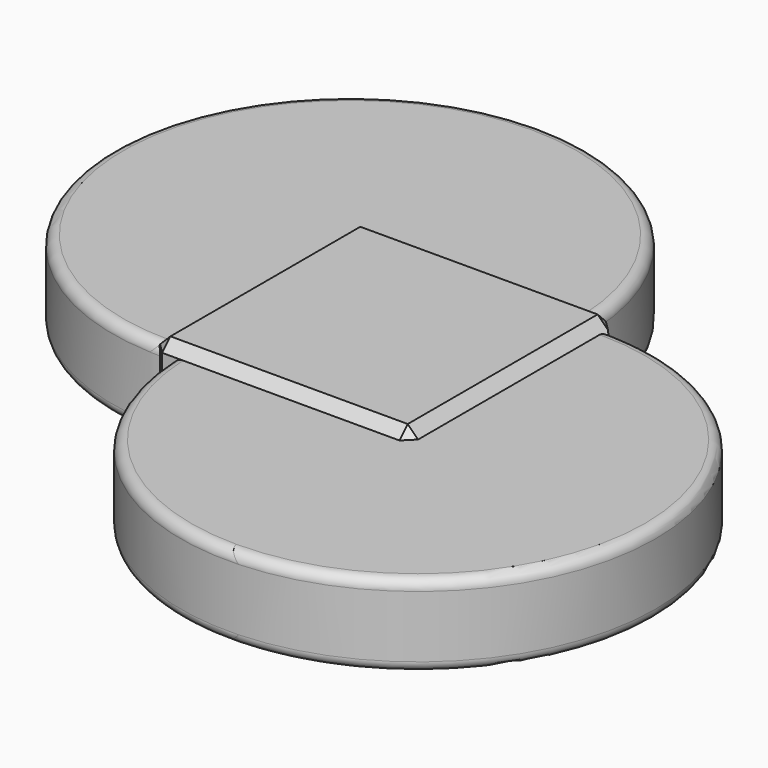
from build123d import *

# Parameters (mm, degrees)
F0_W          = 254
F0_H          = 254
F1_DEPTH      = 50.8
F1_DEPTH_BACK = 50.8
F2_SIZE       = 10.16
F1_FACE_W     = 233.68
F1_FACE_H     = 81.28
F1_FACE1_W    = 233.68
F1_FACE1_H    = 81.28
F5_T4_ANGLE   = 280.0079997231
F5_T9_ANGLE   = 280.0079997231
F5_T14_ANGLE  = 280.0079997231
F5_T19_ANGLE  = 280.0079997231
F5_T24_ANGLE  = 280.0079997231
F5_T29_ANGLE  = 280.0079997231
F5_T34_ANGLE  = 280.0079997231
F5_T39_ANGLE  = 280.0079997231
F5_T44_ANGLE  = 280.0079997231
F5_T49_ANGLE  = 280.0079997231
F5_T54_ANGLE  = 280.0079997231
F5_T59_ANGLE  = 280.0079997231


# Not quite as in the source:
# - a fillet or chamfer that OpenCascade refuses, or shapes differently, is made with other operations: its cross-section is extruded or revolved along the edge and cut away or added


with BuildPart() as f1:
    # F0 (on Top) → F1 (new body, two sides)
    with BuildSketch(Plane.XY) as f1_sk:
        Rectangle(F0_W, F0_H)
    extrude(amount=F1_DEPTH)
    extrude(f1_sk.sketch, amount=-F1_DEPTH_BACK)

    # F2
    f2_edges = [f1.edges().sort_by_distance(p)[0] for p in [
        (0, -127, 50.8),
        (127, -127, 0),
        (127, 0, 50.8),
        (-127, -127, 0),
        (0, -127, -50.8),
        (127, 0, -50.8),
        (127, 127, 0),
        (-127, 0, 50.8),
        (-127, 0, -50.8),
        (-127, 127, 0),
        (0, 127, 50.8),
        (0, 127, -50.8),
    ]]
    chamfer(f2_edges, length=F2_SIZE)

    # F1_face (on face) → F3 (revolve)
    with BuildSketch(Plane.YZ.offset(127)):
        Rectangle(F1_FACE_W, F1_FACE_H)
    revolve(axis=Axis((127, -116.84, 0), (0, 0, -1)))

    # F1_face1 (on face) → F4 (revolve)
    with BuildSketch(Plane(origin=(-127, 0, 0), x_dir=(0, -1, 0), z_dir=(-1, 0, 0))):
        Rectangle(F1_FACE1_W, F1_FACE1_H)
    revolve(axis=Axis((-127, 116.84, 0), (0, 0, 1)))

    # F5: fillet of radius 10.16 on 4 edges, made by hand


with BuildPart() as f5_tool2:
    # F5_s3 → F5_t4 (revolve)
    with BuildSketch(Plane(origin=(112.850510213, 12.3590473355, 0), x_dir=(0, 0, 1), z_dir=(-0.9940564274, -0.1088660602, 0))):
        with BuildLine():
            ThreePointArc((30.48, 103.70845737), (37.6642048969, 100.7326622668), (40.64, 93.54845737))
            Line((40.64, 93.54845737), (40.64, 103.70845737))
            Line((40.64, 103.70845737), (30.48, 103.70845737))
        make_face()
    revolve(axis=Axis((127, -116.84, 40.64), (0, 0, -1)), revolution_arc=F5_T4_ANGLE)

    split(bisect_by=Plane(origin=(83.82, 0, 83.82), x_dir=(0, 1, 0), z_dir=(0.7071067812, 0, 0.7071067812)), keep=Keep.TOP)


with BuildPart() as f1_1:
    add(f1.part)

    # F5_t1: cut F5_tool2
    add(f5_tool2.part, mode=Mode.SUBTRACT)


with BuildPart() as f5_tool7:
    # F5_s8 → F5_t9 (revolve)
    with BuildSketch(Plane(origin=(112.850510213, 12.3590473355, 0), x_dir=(0, 0, 1), z_dir=(-0.9940564274, -0.1088660602, 0))):
        with BuildLine():
            ThreePointArc((30.48, 103.70845737), (37.6642048969, 100.7326622668), (40.64, 93.54845737))
            Line((40.64, 93.54845737), (40.64, 103.70845737))
            Line((40.64, 103.70845737), (30.48, 103.70845737))
        make_face()
    revolve(axis=Axis((127, -116.84, 40.64), (0, 0, -1)), revolution_arc=F5_T9_ANGLE)

    split(bisect_by=Plane(origin=(121.92, 121.92, 0), x_dir=(0, 0, 1), z_dir=(0.7071067812, 0.7071067812, 0)), keep=Keep.TOP)


with BuildPart() as f1_2:
    add(f1_1.part)

    # F5_t6: cut F5_tool7
    add(f5_tool7.part, mode=Mode.SUBTRACT)


with BuildPart() as f5_tool12:
    # F5_s13 → F5_t14 (revolve)
    with BuildSketch(Plane(origin=(112.850510213, 12.3590473355, 0), x_dir=(0, 0, 1), z_dir=(-0.9940564274, -0.1088660602, 0))):
        with BuildLine():
            ThreePointArc((30.48, 103.70845737), (37.6642048969, 100.7326622668), (40.64, 93.54845737))
            Line((40.64, 93.54845737), (40.64, 103.70845737))
            Line((40.64, 103.70845737), (30.48, 103.70845737))
        make_face()
    revolve(axis=Axis((127, -116.84, 40.64), (0, 0, -1)), revolution_arc=F5_T14_ANGLE)

    split(bisect_by=Plane.XZ.offset(127), keep=Keep.TOP)


with BuildPart() as f1_3:
    add(f1_2.part)

    # F5_t11: cut F5_tool12
    add(f5_tool12.part, mode=Mode.SUBTRACT)


with BuildPart() as f5_tool17:
    # F5_s18 → F5_t19 (revolve)
    with BuildSketch(Plane(origin=(112.850510213, 12.3590473355, 0), x_dir=(0, 0, 1), z_dir=(-0.9940564274, -0.1088660602, 0))):
        with BuildLine():
            ThreePointArc((-30.48, 103.70845737), (-37.6642048969, 100.7326622668), (-40.64, 93.54845737))
            Line((-40.64, 93.54845737), (-40.64, 103.70845737))
            Line((-40.64, 103.70845737), (-30.48, 103.70845737))
        make_face()
    revolve(axis=Axis((127, -116.84, -40.64), (0, 0, -1)), revolution_arc=F5_T19_ANGLE)

    split(bisect_by=Plane(origin=(83.82, 0, -83.82), x_dir=(0, 1, 0), z_dir=(0.7071067812, 0, -0.7071067812)), keep=Keep.TOP)


with BuildPart() as f1_4:
    add(f1_3.part)

    # F5_t16: cut F5_tool17
    add(f5_tool17.part, mode=Mode.SUBTRACT)


with BuildPart() as f5_tool22:
    # F5_s23 → F5_t24 (revolve)
    with BuildSketch(Plane(origin=(112.850510213, 12.3590473355, 0), x_dir=(0, 0, 1), z_dir=(-0.9940564274, -0.1088660602, 0))):
        with BuildLine():
            ThreePointArc((-30.48, 103.70845737), (-37.6642048969, 100.7326622668), (-40.64, 93.54845737))
            Line((-40.64, 93.54845737), (-40.64, 103.70845737))
            Line((-40.64, 103.70845737), (-30.48, 103.70845737))
        make_face()
    revolve(axis=Axis((127, -116.84, -40.64), (0, 0, -1)), revolution_arc=F5_T24_ANGLE)

    split(bisect_by=Plane(origin=(121.92, 121.92, 0), x_dir=(0, 0, 1), z_dir=(0.7071067812, 0.7071067812, 0)), keep=Keep.TOP)


with BuildPart() as f1_5:
    add(f1_4.part)

    # F5_t21: cut F5_tool22
    add(f5_tool22.part, mode=Mode.SUBTRACT)


with BuildPart() as f5_tool27:
    # F5_s28 → F5_t29 (revolve)
    with BuildSketch(Plane(origin=(112.850510213, 12.3590473355, 0), x_dir=(0, 0, 1), z_dir=(-0.9940564274, -0.1088660602, 0))):
        with BuildLine():
            ThreePointArc((-30.48, 103.70845737), (-37.6642048969, 100.7326622668), (-40.64, 93.54845737))
            Line((-40.64, 93.54845737), (-40.64, 103.70845737))
            Line((-40.64, 103.70845737), (-30.48, 103.70845737))
        make_face()
    revolve(axis=Axis((127, -116.84, -40.64), (0, 0, -1)), revolution_arc=F5_T29_ANGLE)

    split(bisect_by=Plane.XZ.offset(127), keep=Keep.TOP)


with BuildPart() as f1_6:
    add(f1_5.part)

    # F5_t26: cut F5_tool27
    add(f5_tool27.part, mode=Mode.SUBTRACT)


with BuildPart() as f5_tool32:
    # F5_s33 → F5_t34 (revolve)
    with BuildSketch(Plane(origin=(7.0960267411, 108.0319683984, 0), x_dir=(0, 0, 1), z_dir=(-0.0655432689, -0.9978497281, 0))):
        with BuildLine():
            ThreePointArc((-30.48, -99.2950089912), (-37.6642048969, -96.319213888), (-40.64, -89.1350089912))
            Line((-40.64, -89.1350089912), (-40.64, -99.2950089912))
            Line((-40.64, -99.2950089912), (-30.48, -99.2950089912))
        make_face()
    revolve(axis=Axis((-127, 116.84, -40.64), (0, 0, 1)), revolution_arc=F5_T34_ANGLE)

    split(bisect_by=Plane.XZ.offset(-127), keep=Keep.BOTTOM)


with BuildPart() as f1_7:
    add(f1_6.part)

    # F5_t31: cut F5_tool32
    add(f5_tool32.part, mode=Mode.SUBTRACT)


with BuildPart() as f5_tool37:
    # F5_s38 → F5_t39 (revolve)
    with BuildSketch(Plane(origin=(7.0960267411, 108.0319683984, 0), x_dir=(0, 0, 1), z_dir=(-0.0655432689, -0.9978497281, 0))):
        with BuildLine():
            ThreePointArc((-30.48, -99.2950089912), (-37.6642048969, -96.319213888), (-40.64, -89.1350089912))
            Line((-40.64, -89.1350089912), (-40.64, -99.2950089912))
            Line((-40.64, -99.2950089912), (-30.48, -99.2950089912))
        make_face()
    revolve(axis=Axis((-127, 116.84, -40.64), (0, 0, 1)), revolution_arc=F5_T39_ANGLE)

    split(bisect_by=Plane(origin=(-83.82, 0, -83.82), x_dir=(0, 1, 0), z_dir=(-0.7071067812, 0, -0.7071067812)), keep=Keep.TOP)


with BuildPart() as f1_8:
    add(f1_7.part)

    # F5_t36: cut F5_tool37
    add(f5_tool37.part, mode=Mode.SUBTRACT)


with BuildPart() as f5_tool42:
    # F5_s43 → F5_t44 (revolve)
    with BuildSketch(Plane(origin=(7.0960267411, 108.0319683984, 0), x_dir=(0, 0, 1), z_dir=(-0.0655432689, -0.9978497281, 0))):
        with BuildLine():
            ThreePointArc((-30.48, -99.2950089912), (-37.6642048969, -96.319213888), (-40.64, -89.1350089912))
            Line((-40.64, -89.1350089912), (-40.64, -99.2950089912))
            Line((-40.64, -99.2950089912), (-30.48, -99.2950089912))
        make_face()
    revolve(axis=Axis((-127, 116.84, -40.64), (0, 0, 1)), revolution_arc=F5_T44_ANGLE)

    split(bisect_by=Plane(origin=(-121.92, -121.92, 0), x_dir=(0, 0, 1), z_dir=(-0.7071067812, -0.7071067812, 0)), keep=Keep.TOP)


with BuildPart() as f1_9:
    add(f1_8.part)

    # F5_t41: cut F5_tool42
    add(f5_tool42.part, mode=Mode.SUBTRACT)


with BuildPart() as f5_tool47:
    # F5_s48 → F5_t49 (revolve)
    with BuildSketch(Plane(origin=(7.0960267411, 108.0319683984, 0), x_dir=(0, 0, 1), z_dir=(-0.0655432689, -0.9978497281, 0))):
        with BuildLine():
            ThreePointArc((30.48, -99.2950089912), (37.6642048969, -96.319213888), (40.64, -89.1350089912))
            Line((40.64, -89.1350089912), (40.64, -99.2950089912))
            Line((40.64, -99.2950089912), (30.48, -99.2950089912))
        make_face()
    revolve(axis=Axis((-127, 116.84, 40.64), (0, 0, 1)), revolution_arc=F5_T49_ANGLE)

    split(bisect_by=Plane.XZ.offset(-127), keep=Keep.BOTTOM)


with BuildPart() as f1_10:
    add(f1_9.part)

    # F5_t46: cut F5_tool47
    add(f5_tool47.part, mode=Mode.SUBTRACT)


with BuildPart() as f5_tool52:
    # F5_s53 → F5_t54 (revolve)
    with BuildSketch(Plane(origin=(7.0960267411, 108.0319683984, 0), x_dir=(0, 0, 1), z_dir=(-0.0655432689, -0.9978497281, 0))):
        with BuildLine():
            ThreePointArc((30.48, -99.2950089912), (37.6642048969, -96.319213888), (40.64, -89.1350089912))
            Line((40.64, -89.1350089912), (40.64, -99.2950089912))
            Line((40.64, -99.2950089912), (30.48, -99.2950089912))
        make_face()
    revolve(axis=Axis((-127, 116.84, 40.64), (0, 0, 1)), revolution_arc=F5_T54_ANGLE)

    split(bisect_by=Plane(origin=(-83.82, 0, 83.82), x_dir=(0, 1, 0), z_dir=(-0.7071067812, 0, 0.7071067812)), keep=Keep.TOP)


with BuildPart() as f1_11:
    add(f1_10.part)

    # F5_t51: cut F5_tool52
    add(f5_tool52.part, mode=Mode.SUBTRACT)


with BuildPart() as f5_tool57:
    # F5_s58 → F5_t59 (revolve)
    with BuildSketch(Plane(origin=(7.0960267411, 108.0319683984, 0), x_dir=(0, 0, 1), z_dir=(-0.0655432689, -0.9978497281, 0))):
        with BuildLine():
            ThreePointArc((30.48, -99.2950089912), (37.6642048969, -96.319213888), (40.64, -89.1350089912))
            Line((40.64, -89.1350089912), (40.64, -99.2950089912))
            Line((40.64, -99.2950089912), (30.48, -99.2950089912))
        make_face()
    revolve(axis=Axis((-127, 116.84, 40.64), (0, 0, 1)), revolution_arc=F5_T59_ANGLE)

    split(bisect_by=Plane(origin=(-121.92, -121.92, 0), x_dir=(0, 0, 1), z_dir=(-0.7071067812, -0.7071067812, 0)), keep=Keep.TOP)


with BuildPart() as f1_12:
    add(f1_11.part)

    # F5_t56: cut F5_tool57
    add(f5_tool57.part, mode=Mode.SUBTRACT)


solid = f1_12.part
